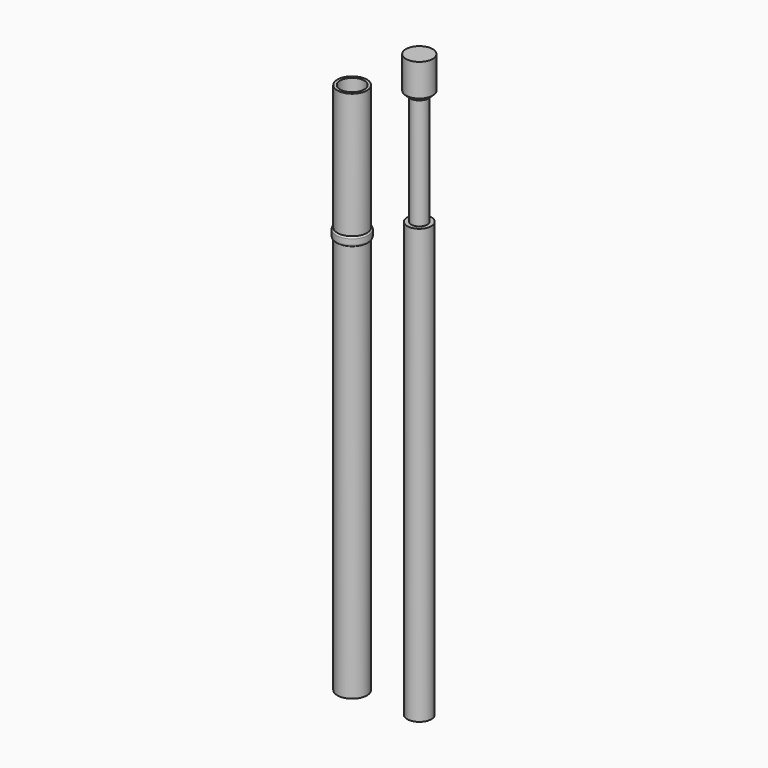
from build123d import *

# Parameters (mm, degrees)
F0_R     = 0.84
F0_R_2   = 0.685
F1_DEPTH = 30.23
F2_R     = 0.685
F3_DEPTH = 24.64
F4_R     = 0.455
F5_DEPTH = 6.35
F6_R     = 0.76
F7_DEPTH = 2.03
F8_SIZE  = 0.2
F9_W     = 0.915
F9_H     = 0.5


# Not quite as in the source:
# - a fillet or chamfer that OpenCascade refuses, or shapes differently, is made with other operations: its cross-section is extruded or revolved along the edge and cut away or added


with BuildPart() as f1:
    # F0 (on Top) → F1 (new body)
    with BuildSketch(Plane.XY):
        Circle(F0_R)
        Circle(F0_R_2, mode=Mode.SUBTRACT)
    extrude(amount=F1_DEPTH)

    # F9 (on Front) → F10 (revolve)
    with BuildSketch(Plane.XZ):
        with Locations((-0.4575, 22.86)):
            Rectangle(F9_W, F9_H)
    revolve(axis=Axis((0, 0, 22.86), (0, 0, -1)))

    # F11: fillet of radius 0.1 on 2 edges, made by hand

    # F11_s1 → F11_t2 (revolve, cut)
    with BuildSketch(Plane.XZ):
        with BuildLine():
            ThreePointArc((-0.915, 23.0131754163), (-0.8940569415, 23.0744126599), (-0.84, 23.11))
            Line((-0.84, 23.11), (-0.915, 23.11))
            Line((-0.915, 23.11), (-0.915, 23.0131754163))
        make_face()
    revolve(axis=Axis((0, 0, 23.11), (0, 0, -1)), mode=Mode.SUBTRACT)

    # F11_s3 → F11_t4 (revolve, cut)
    with BuildSketch(Plane.XZ):
        with BuildLine():
            ThreePointArc((-0.84, 22.61), (-0.8940569415, 22.6455873401), (-0.915, 22.7068245837))
            Line((-0.915, 22.7068245837), (-0.915, 22.61))
            Line((-0.915, 22.61), (-0.84, 22.61))
        make_face()
    revolve(axis=Axis((0, 0, 22.61), (0, 0, -1)), mode=Mode.SUBTRACT)


with BuildPart() as f3:
    # F2 (on Top) → F3 (new body)
    with BuildSketch(Plane.XY):
        with Locations((3.8109193556, 0)):
            Circle(F2_R)
    extrude(amount=F3_DEPTH)

    # F4 (on face) → F5 (join)
    with BuildSketch(Plane.XY.offset(24.64)):
        with Locations((3.8109193556, 0)):
            Circle(F4_R)
    extrude(amount=F5_DEPTH)

    # F6 (on face) → F7 (join)
    with BuildSketch(Plane.XY.offset(30.99)):
        with Locations((3.8109193556, 0)):
            Circle(F6_R)
    extrude(amount=F7_DEPTH)

    # F8
    f8_edges = [f3.edges().sort_by_distance(p)[0] for p in [
        (3.050919, 0, 30.99),
    ]]
    chamfer(f8_edges, length=F8_SIZE)


solid = Compound([f1.part, f3.part])
